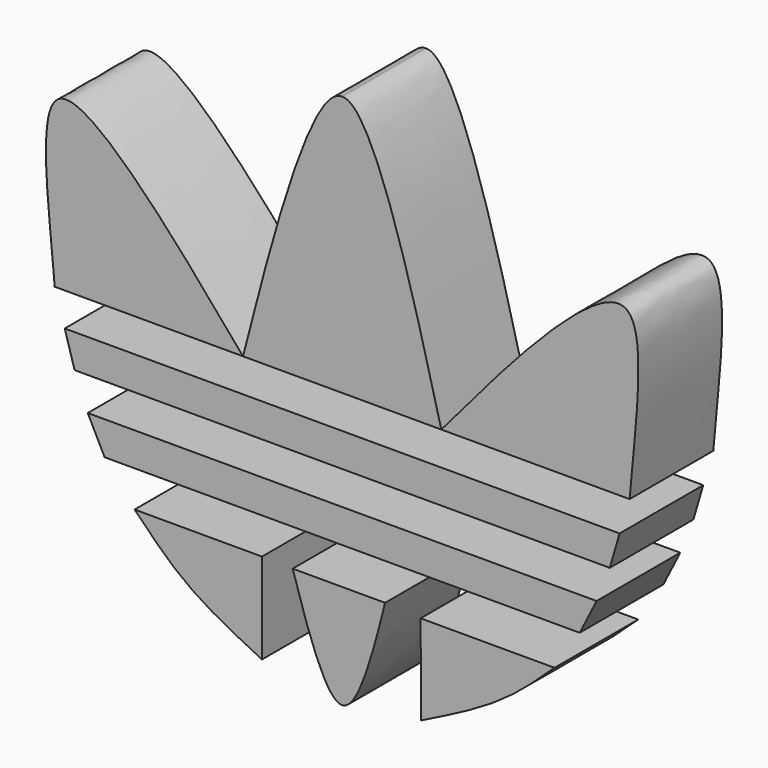
from build123d import *

# Parameters (mm, degrees)
F1_DEPTH = 25


with BuildPart() as f1:
    # F0 (on Front) → F1 (new body)
    with BuildSketch(Plane.XZ):
        with BuildLine():
            Line((-68.6997125745, 0), (-23.6997125745, 0))
            add(Edge.make_bspline(
                [(-23.6997125745, 0), (-39.0522736523, 18.2610777884), (-77.4283213345, 63.5335866827), (-69.9814380991, 15.9987635125), (-68.6997125745, 0)],
                knots=[0, 0, 0, 0, 0.5488298185, 1, 1, 1, 1], degree=3))
        make_face()
    extrude(amount=F1_DEPTH)


with BuildPart() as f1b:
    # F0 (on Front) → F1, piece 2 (new body)
    with BuildSketch(Plane.XZ):
        with BuildLine():
            add(Edge.make_bspline(
                [(-23.6997125745, 0), (-15.7709243038, 31.3297332335), (-7.0324667798, 62.6286994315), (-1.17e-08, 62.3443424706)],
                knots=[0, 0, 0, 0, 0.5032701678, 0.5032701678, 0.5032701678, 0.5032701678], degree=3))
            Line((-23.6997125745, 0), (-18.3002874255, 0))
            add(Edge.make_bspline(
                [(-1.17e-08, 62.3443424697), (-6.9410751237, 62.0636808676), (-12.2202123623, 31.0152552891), (-18.3002874255, 0)],
                knots=[0.5032701678, 0.5032701678, 0.5032701678, 0.5032701678, 1, 1, 1, 1], degree=3))
        make_face()
        with BuildLine():
            add(Edge.make_bspline(
                [(-1.17e-08, 62.3443424697), (-6.9410751237, 62.0636808676), (-12.2202123623, 31.0152552891), (-18.3002874255, 0)],
                knots=[0.5032701678, 0.5032701678, 0.5032701678, 0.5032701678, 1, 1, 1, 1], degree=3))
            Line((-18.3002874255, 0), (0, 0))
            Line((0, 0), (18.3002874255, 0))
            add(Edge.make_bspline(
                [(-1.17e-08, 62.3443424706), (6.9410751148, 62.06368092), (12.2202123623, 31.0152552891), (18.3002874255, 0)],
                knots=[0.5032701678, 0.5032701678, 0.5032701678, 0.5032701678, 1, 1, 1, 1], degree=3))
        make_face()
        with BuildLine():
            add(Edge.make_bspline(
                [(23.6997125745, 0), (15.7709243038, 31.3297332335), (7.0324667652, 62.6286994836), (-1.17e-08, 62.3443424697)],
                knots=[0, 0, 0, 0, 0.5032701678, 0.5032701678, 0.5032701678, 0.5032701678], degree=3))
            add(Edge.make_bspline(
                [(-1.17e-08, 62.3443424706), (6.9410751148, 62.06368092), (12.2202123623, 31.0152552891), (18.3002874255, 0)],
                knots=[0.5032701678, 0.5032701678, 0.5032701678, 0.5032701678, 1, 1, 1, 1], degree=3))
            Line((18.3002874255, 0), (23.6997125745, 0))
        make_face()
    extrude(amount=F1_DEPTH)


with BuildPart() as f1c:
    # F0 (on Front) → F1, piece 3 (new body)
    with BuildSketch(Plane.XZ):
        with BuildLine():
            add(Edge.make_bspline(
                [(23.6997125745, 0), (39.0522736523, 18.2610777884), (77.4283213345, 63.5335866827), (69.9814380991, 15.9987635125), (68.6997125745, 0)],
                knots=[0, 0, 0, 0, 0.5488298185, 1, 1, 1, 1], degree=3))
            Line((23.6997125745, 0), (68.6997125745, 0))
        make_face()
    extrude(amount=F1_DEPTH)


with BuildPart() as f1d:
    # F0 (on Front) → F1, piece 4 (new body)
    with BuildSketch(Plane.XZ):
        Polygon((0, -8), (-66.3058993968, -8), (-63.9578328955, -16), (0, -16), (63.9578328955, -16), (66.3058993968, -8), align=None)
    extrude(amount=F1_DEPTH)


with BuildPart() as f1e:
    # F0 (on Front) → F1, piece 5 (new body)
    with BuildSketch(Plane.XZ):
        Polygon((0, -24), (-60.8107628588, -24), (-56.7733727334, -32), (0, -32), (56.7733727334, -32), (60.8107628588, -24), align=None)
    extrude(amount=F1_DEPTH)


with BuildPart() as f1f:
    # F0 (on Front) → F1, piece 6 (new body)
    with BuildSketch(Plane.XZ):
        with BuildLine():
            Line((-19.1602188304, -40.6652976506), (-49.6079055849, -40.6652976506))
            add(Edge.make_bspline(
                [(-49.6079055849, -40.6652976506), (-45.6042762075, -44.7987540399), (-37.323531991, -53.42044232), (-25.350073964, -59.2691873867), (-19.1602188304, -62.3217699111)],
                knots=[0, 0, 0, 0, 0.4817230649, 1, 1, 1, 1], degree=3))
            Line((-19.1602188304, -62.3217699111), (-19.1602188304, -40.6652976506))
        make_face()
    extrude(amount=F1_DEPTH)


with BuildPart() as f1g:
    # F0 (on Front) → F1, piece 7 (new body)
    with BuildSketch(Plane.XZ):
        with BuildLine():
            add(Edge.make_bspline(
                [(50.7549608034, -41.3243134417), (46.6897149867, -45.1485426126), (38.0826848799, -53.2794044405), (25.4981687947, -59.4868820492), (18.8551553599, -62.7781776149)],
                knots=[0, 0, 0, 0, 0.471510682, 1, 1, 1, 1], degree=3))
            Line((50.7549608034, -41.3243134417), (18.7549608034, -41.3243134417))
            Line((18.7549608034, -41.3243134417), (18.8551553599, -62.7781776149))
        make_face()
    extrude(amount=F1_DEPTH)


with BuildPart() as f1h:
    # F0 (on Front) → F1, piece 8 (new body)
    with BuildSketch(Plane.XZ):
        with BuildLine():
            Line((10.2589651942, -40.8205576241), (-11.8273422122, -40.8205576241))
            add(Edge.make_bspline(
                [(-11.8273422122, -40.8205576241), (-7.7598916227, -54.2035082505), (0.3132963291, -77.2394406177), (6.9613261908, -54.0939511769), (10.2589651942, -40.8205576241)],
                knots=[0, 0, 0, 0, 0.5029213178, 1, 1, 1, 1], degree=3))
        make_face()
    extrude(amount=F1_DEPTH)


solid = Compound([f1.part, f1b.part, f1c.part, f1d.part, f1e.part, f1f.part, f1g.part, f1h.part])
